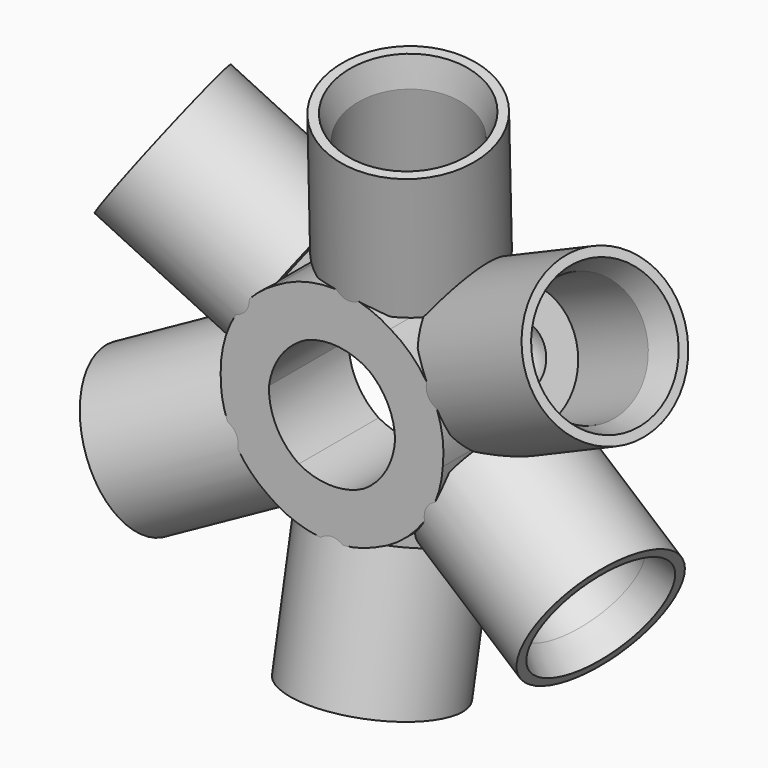
from build123d import *

# Parameters (mm, degrees)
F0_R          = 23.5
F0_R_2        = 15
F4_DEPTH      = 18
F4_DEPTH_BACK = 4
F6_COUNT      = 2
F6_ANGLE      = 63.25
F7_COUNT      = 2
F7_ANGLE      = 61.5
F8_COUNT      = 2
F8_ANGLE      = 116.5
F9_COUNT      = 2
F9_ANGLE      = 188
F10_COUNT     = 2
F10_ANGLE     = 126.5
F13_TEXT_SIZE = 10.5029541171
F14_DEPTH     = 2


# Not quite as in the source:
# - Text() gives the source's letters only with a copy of the font that has no kerning and outlines rounded to 1/6400 em; it was checked with that copy


with BuildPart() as f3:
    # F2 (on line) → F3 (revolve)
    with BuildSketch(Plane(origin=(0, -3.7526447404, 0.7464474492), x_dir=(1, 0, 0), z_dir=(0, -0.9807852804, 0.195090322))):
        with BuildLine():
            Line((6.7275495715, 11.1909703114), (13.39, 11.1909703114))
            Line((13.39, 11.1909703114), (13.39, -10.2532064901))
            Line((13.39, -10.2532064901), (15.39, -16.5995957263))
            Line((15.39, -16.5995957263), (17.39, -16.5995957263))
            Line((17.39, -16.5995957263), (17.39, 15.1909703114))
            Line((17.39, 15.1909703114), (8.4690514833, 15.1909703114))
            ThreePointArc((8.4690514833, 15.1909703114), (5.0129940493, 19.1026530457), (0, 20.557123899))
            Line((0, 20.557123899), (0, 17.9185198829))
            ThreePointArc((0, 17.9185198829), (4.7570959228, 15.9480662342), (6.7275495715, 11.1909703114))
        make_face()
    revolve(axis=Axis((0, 0.0004681272, 19.6146199869), (0, 0.195090322, 0.9807852804)))

    # F0 (on Front) → F4 (join, two sides)
    with BuildSketch(Plane.XZ) as f4_sk:
        with Locations((0, 43.1122665526)):
            Circle(F0_R)
        with Locations((0, 43.1122665526)):
            Circle(F0_R_2, mode=Mode.SUBTRACT)
    extrude(amount=F4_DEPTH)
    extrude(f4_sk.sketch, amount=-F4_DEPTH_BACK)


with BuildPart() as f6_1:
    # F6: instance of F3
    add(f3.part.rotate(Axis((0, -4.9195094034, 41.8967977166), (0, 1, 0)), 1 * F6_ANGLE / (F6_COUNT - 1)))


with BuildPart() as f7_1:
    # F7: instance of F3
    add(f3.part.rotate(Axis((0, -4.9195094034, 41.8967977166), (0, -1, 0)), 1 * F7_ANGLE / (F7_COUNT - 1)))


with BuildPart() as f8_1:
    # F8: instance of F3
    add(f3.part.rotate(Axis((0, -4.9195094034, 41.8967977166), (0, -1, 0)), 1 * F8_ANGLE / (F8_COUNT - 1)))


with BuildPart() as f9_1:
    # F9: instance of F3
    add(f3.part.rotate(Axis((0, -4.9195094034, 41.8967977166), (0, 1, 0)), 1 * F9_ANGLE / (F9_COUNT - 1)))


with BuildPart() as f10_1:
    # F10: instance of F3
    add(f3.part.rotate(Axis((0, -4.9195094034, 41.8967977166), (0, 1, 0)), 1 * F10_ANGLE / (F10_COUNT - 1)))


with BuildPart() as f3_1:
    add(f3.part)

    # F11: union F6_1, F8_1, F9_1, F10_1, F7_1
    add(f6_1.part)
    add(f8_1.part)
    add(f9_1.part)
    add(f10_1.part)
    add(f7_1.part)

    # F13 (on offset) → F14 (join)
    with BuildSketch(Plane(origin=(0, 4, 0), x_dir=(-1, 0, 0), z_dir=(0, 1, 0))):
        with Locations((-19.0558712929, 47.8909797966)):
            Text('G', F13_TEXT_SIZE, font='Open Sans', text_align=(TextAlign.LEFT, TextAlign.BOTTOM))
    extrude(amount=F14_DEPTH)


solid = f3_1.part
